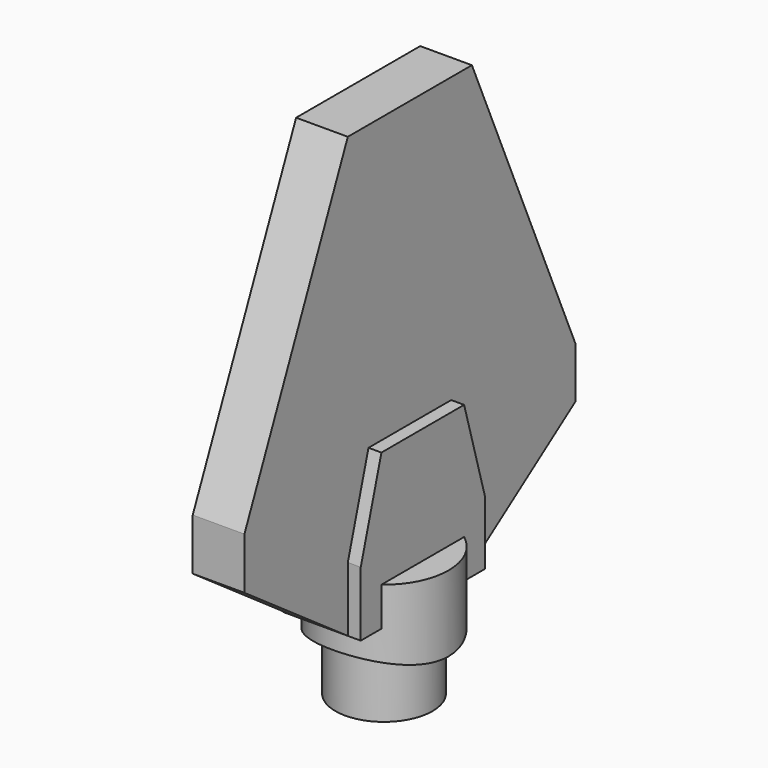
from build123d import *

# Parameters (mm, degrees)
F0_R         = 5
F1_DEPTH     = 6
F3_R         = 15
F4_DEPTH     = 25
F5_R         = 3.75
F6_DEPTH     = 10
F8_DEPTH     = 2
F9_DEPTH     = 2
F10_T1_DEPTH = 55.6511992514
F11_T1_DEPTH = 55.6511992514
F12_SIZE2    = 23
F12_SIZE     = 10
F14_W        = 12
F14_H        = 12
F15_DEPTH    = 1
F16_W        = 12
F16_H        = 12
F17_DEPTH    = 1
F18_SIZE2    = 7
F18_SIZE     = 2
F19_SIZE2    = 7
F19_SIZE     = 2


# Not quite as in the source:
# - a fillet or chamfer that OpenCascade refuses, or shapes differently, is made with other operations: its cross-section is extruded or revolved along the edge and cut away or added
# - two fillets or chamfers of one size are made in one step


with BuildPart() as f1:
    # F0 (on Top) → F1 (new body)
    with BuildSketch(Plane.XY):
        Circle(F0_R)
    extrude(amount=F1_DEPTH)

    # F3 (on offset) → F4 (cut)
    with BuildSketch(Plane.XZ.offset(6)):
        with Locations((0, -14)):
            Circle(F3_R)
    extrude(amount=-F4_DEPTH, mode=Mode.SUBTRACT)

    # F5 (on face) → F6 (join)
    with BuildSketch(Plane.XY.offset(6)):
        Circle(F5_R)
    extrude(amount=-F6_DEPTH)

    # F7 (on Right) → F8 (join)
    with BuildSketch(Plane.YZ):
        Polygon((16, 3), (16, 37), (-16, 37), (-16, 3), (0, 3), align=None)
    extrude(amount=F8_DEPTH)

    # F9 (add): a face of the model
    f9_faces = [f1.faces().sort_by_distance(p)[0] for p in [
        (0, 0, 20.4395085066),
    ]]
    extrude(f9_faces, amount=F9_DEPTH)

    # F10: chamfer of 10 x 7 on 1 edges, made by hand

    # F10_s2 → F10_t1 (cut)
    with BuildSketch(Plane.YZ.offset(-27.8255996257)):
        Polygon((-16, 10), (-6, 3), (-16, 3), align=None)
    extrude(amount=F10_T1_DEPTH, mode=Mode.SUBTRACT)

    # F11: chamfer of 7 x 10 on 1 edges, made by hand

    # F11_s2 → F11_t1 (cut)
    with BuildSketch(Plane.YZ.offset(-27.8255996257)):
        Polygon((6, 3), (16, 10), (16, 3), align=None)
    extrude(amount=F11_T1_DEPTH, mode=Mode.SUBTRACT)

    # F12
    f12_edges = [f1.edges().sort_by_distance(p)[0] for p in [
        (0, -16, 37),
        (0, 16, 37),
    ]]
    f12_side = f1.faces().sort_by_distance((0, 0, 37))[0]
    chamfer(f12_edges, length=F12_SIZE, length2=F12_SIZE2, reference=f12_side)

    # F14 (on face) → F15 (join)
    with BuildSketch(Plane(origin=(-2, 0, 0), x_dir=(0, -1, 0), z_dir=(-1, 0, 0))):
        with Locations((0, 9)):
            Rectangle(F14_W, F14_H)
    extrude(amount=F15_DEPTH)

    # F16 (on face) → F17 (join)
    with BuildSketch(Plane.YZ.offset(2)):
        with Locations((0, 9)):
            Rectangle(F16_W, F16_H)
    extrude(amount=F17_DEPTH)

    # F18
    f18_edges = [f1.edges().sort_by_distance(p)[0] for p in [
        (-2.5, -6, 15),
        (-2.5, 6, 15),
    ]]
    f18_side = f1.faces().sort_by_distance((-2.5, 0, 15))[0]
    chamfer(f18_edges, length=F18_SIZE, length2=F18_SIZE2, reference=f18_side)

    # F19
    f19_edges = [f1.edges().sort_by_distance(p)[0] for p in [
        (2.5, 6, 15),
        (2.5, -6, 15),
    ]]
    f19_side = f1.faces().sort_by_distance((2.5, 0, 15))[0]
    chamfer(f19_edges, length=F19_SIZE, length2=F19_SIZE2, reference=f19_side)


solid = f1.part
